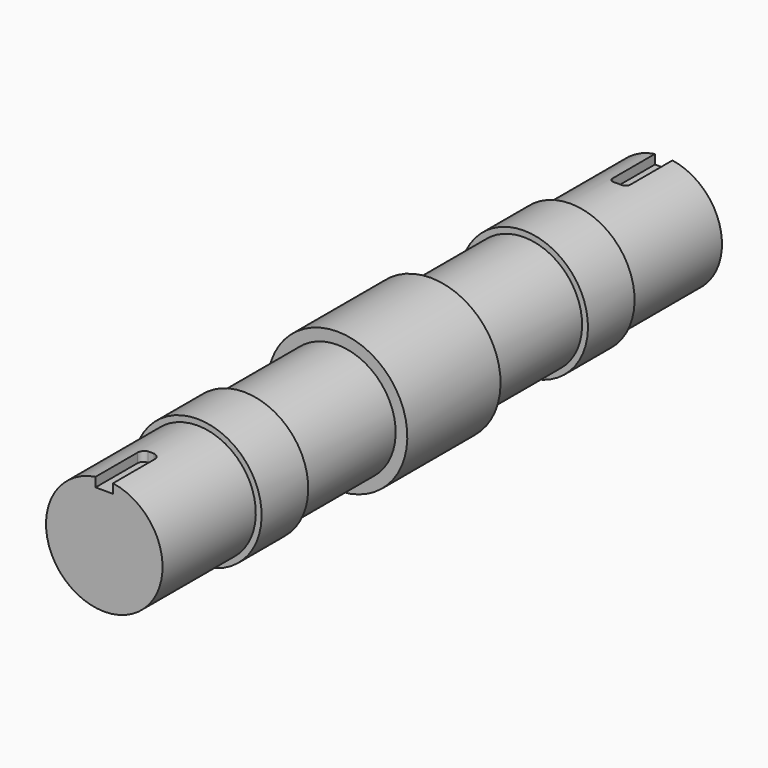
from build123d import *

# Parameters (mm, degrees)
F3_DEPTH = 50
F4_R     = 5


# Not quite as in the source:
# - a pattern or mirror of a feature is missing from the dataset's text; its kind, count and spacing are read off the source's solid


with BuildPart() as f1:
    # F0 (on Right) → F1 (revolve)
    with BuildSketch(Plane.YZ):
        Polygon((-300, 50), (-300, 0), (300, 0), (300, 50), (200, 50), (200, 55), (150, 55), (150, 50), (50, 50), (50, 60), (-50, 60), (-50, 50), (-150, 50), (-150, 55), (-200, 55), (-200, 50), align=None)
    revolve(axis=Axis((0, 0, 0), (0, 1, 0)))

    # F2 (on face) → F3 (cut)
    with BuildSketch(Plane.XZ.offset(300)):
        with BuildLine():
            Line((-7.5, 41.4342998332), (7.5, 41.4342998332))
            Line((7.5, 41.4342998332), (7.5, 49.4342998332))
            ThreePointArc((7.5, 49.4342998332), (0, 50), (-7.5, 49.4342998332))
            Line((-7.5, 49.4342998332), (-7.5, 41.4342998332))
        make_face()
    f3 = extrude(amount=-F3_DEPTH, mode=Mode.SUBTRACT)

    # F3_copies: F3 across plane
    add(f3.mirror(Plane.ZX), mode=Mode.SUBTRACT)

    # F4
    f4_edges = [f1.edges().sort_by_distance(p)[0] for p in [
        (-7.5, -250, 45.4343),
        (7.5, -250, 45.4343),
        (7.5, 250, 45.4343),
        (-7.5, 250, 45.4343),
    ]]
    fillet(f4_edges, radius=F4_R)


solid = f1.part
